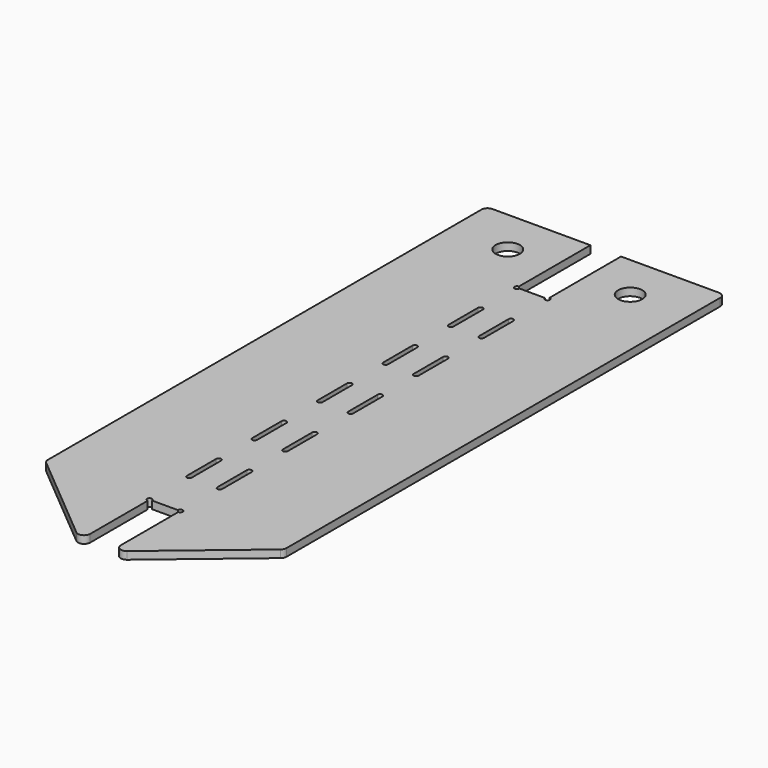
from build123d import *

# Parameters (mm, degrees)
F0_R     = 2.50825
F1_DEPTH = 1.5875
F2_R     = 1.27


with BuildPart() as f1:
    # F0 (on Top) → F1 (new body)
    with BuildSketch(Plane.XY):
        with BuildLine():
            Line((2.667, 95.25), (0, 95.25))
            Line((0, 95.25), (-2.667, 95.25))
            ThreePointArc((-2.667, 95.25), (-3.5342102448, 94.8907897552), (-3.175, 95.758))
            Line((-3.175, 95.758), (-3.175, 114.3))
            Line((-3.175, 114.3), (-24.765, 114.3))
            Line((-24.765, 114.3), (-24.765, 0))
            Line((-24.765, 0), (-5.2613402643, -16.3655136908))
            ThreePointArc((-5.2613402643, -16.3655136908), (-3.9082748076, -16.5436481376), (-3.175, -15.3926372481))
            Line((-3.175, -15.3926372481), (-3.175, -0.508))
            ThreePointArc((-3.175, -0.508), (-3.5342102448, 0.3592102448), (-2.667, 0))
            Line((-2.667, 0), (0, 0))
            Line((0, 0), (2.667, 0))
            ThreePointArc((2.667, 0), (3.3487462328, 0.4773638514), (3.5641505771, -0.3265361057))
            ThreePointArc((3.5641505771, -0.3265361057), (3.389690077, -0.4604043558), (3.175, -0.508))
            Line((3.175, -0.508), (3.175, -15.3926372481))
            ThreePointArc((3.175, -15.3926372481), (3.9082748076, -16.5436481376), (5.2613402643, -16.3655136908))
            Line((5.2613402643, -16.3655136908), (24.765, 0))
            Line((24.765, 0), (24.765, 114.3))
            Line((24.765, 114.3), (3.175, 114.3))
            Line((3.175, 114.3), (3.175, 95.758))
            ThreePointArc((3.175, 95.758), (3.5342102448, 94.8907897552), (2.667, 95.25))
        make_face()
        with BuildLine():
            ThreePointArc((-3.683, 17.8998578738), (-3.175, 18.4078578738), (-2.667, 17.8998578738))
            Line((-2.667, 17.8998578738), (-2.667, 10.2798578738))
            ThreePointArc((-2.667, 10.2798578738), (-3.175, 9.7718578738), (-3.683, 10.2798578738))
            Line((-3.683, 10.2798578738), (-3.683, 17.8998578738))
        make_face(mode=Mode.SUBTRACT)
        with BuildLine():
            ThreePointArc((-3.683, 34.8687778738), (-3.175, 35.3767778738), (-2.667, 34.8687778738))
            Line((-2.667, 34.8687778738), (-2.667, 27.2487778738))
            ThreePointArc((-2.667, 27.2487778738), (-3.175, 26.7407778738), (-3.683, 27.2487778738))
            Line((-3.683, 27.2487778738), (-3.683, 34.8687778738))
        make_face(mode=Mode.SUBTRACT)
        with BuildLine():
            Line((-3.683, 44.2176978738), (-3.683, 51.8376978738))
            ThreePointArc((-3.683, 51.8376978738), (-3.175, 52.3456978738), (-2.667, 51.8376978738))
            Line((-2.667, 51.8376978738), (-2.667, 44.2176978738))
            ThreePointArc((-2.667, 44.2176978738), (-3.175, 43.7096978738), (-3.683, 44.2176978738))
        make_face(mode=Mode.SUBTRACT)
        with BuildLine():
            Line((3.683, 17.8998578738), (3.683, 10.2798578738))
            ThreePointArc((3.683, 10.2798578738), (3.175, 9.7718578738), (2.667, 10.2798578738))
            Line((2.667, 10.2798578738), (2.667, 17.8998578738))
            ThreePointArc((2.667, 17.8998578738), (3.175, 18.4078578738), (3.683, 17.8998578738))
        make_face(mode=Mode.SUBTRACT)
        with BuildLine():
            Line((3.683, 34.8687778738), (3.683, 27.2487778738))
            ThreePointArc((3.683, 27.2487778738), (3.175, 26.7407778738), (2.667, 27.2487778738))
            Line((2.667, 27.2487778738), (2.667, 34.8687778738))
            ThreePointArc((2.667, 34.8687778738), (3.175, 35.3767778738), (3.683, 34.8687778738))
        make_face(mode=Mode.SUBTRACT)
        with BuildLine():
            Line((3.683, 51.8376978738), (3.683, 44.2176978738))
            ThreePointArc((3.683, 44.2176978738), (3.175, 43.7096978738), (2.667, 44.2176978738))
            Line((2.667, 44.2176978738), (2.667, 51.8376978738))
            ThreePointArc((2.667, 51.8376978738), (3.175, 52.3456978738), (3.683, 51.8376978738))
        make_face(mode=Mode.SUBTRACT)
        with BuildLine():
            ThreePointArc((-3.683, 68.8048978738), (-3.175, 69.3128978738), (-2.667, 68.8048978738))
            Line((-2.667, 68.8048978738), (-2.667, 61.1848978738))
            ThreePointArc((-2.667, 61.1848978738), (-3.175, 60.6768978738), (-3.683, 61.1848978738))
            Line((-3.683, 61.1848978738), (-3.683, 68.8048978738))
        make_face(mode=Mode.SUBTRACT)
        with Locations((-12.7, 104.775)):
            Circle(F0_R, mode=Mode.SUBTRACT)
        with BuildLine():
            ThreePointArc((-3.683, 85.7720978738), (-3.175, 86.2800978738), (-2.667, 85.7720978738))
            Line((-2.667, 85.7720978738), (-2.667, 78.1520978738))
            ThreePointArc((-2.667, 78.1520978738), (-3.175, 77.6440978738), (-3.683, 78.1520978738))
            Line((-3.683, 78.1520978738), (-3.683, 85.7720978738))
        make_face(mode=Mode.SUBTRACT)
        with BuildLine():
            Line((3.683, 68.8048978738), (3.683, 61.1848978738))
            ThreePointArc((3.683, 61.1848978738), (3.175, 60.6768978738), (2.667, 61.1848978738))
            Line((2.667, 61.1848978738), (2.667, 68.8048978738))
            ThreePointArc((2.667, 68.8048978738), (3.175, 69.3128978738), (3.683, 68.8048978738))
        make_face(mode=Mode.SUBTRACT)
        with BuildLine():
            Line((3.683, 85.7720978738), (3.683, 78.1520978738))
            ThreePointArc((3.683, 78.1520978738), (3.175, 77.6440978738), (2.667, 78.1520978738))
            Line((2.667, 78.1520978738), (2.667, 85.7720978738))
            ThreePointArc((2.667, 85.7720978738), (3.175, 86.2800978738), (3.683, 85.7720978738))
        make_face(mode=Mode.SUBTRACT)
        with Locations((12.7, 104.775)):
            Circle(F0_R, mode=Mode.SUBTRACT)
    extrude(amount=F1_DEPTH)

    # F2
    f2_edges = [f1.edges().sort_by_distance(p)[0] for p in [
        (24.765, 0, 0.79375),
        (-24.765, 0, 0.79375),
        (-24.765, 114.3, 0.79375),
        (24.765, 114.3, 0.79375),
    ]]
    fillet(f2_edges, radius=F2_R)


solid = f1.part
